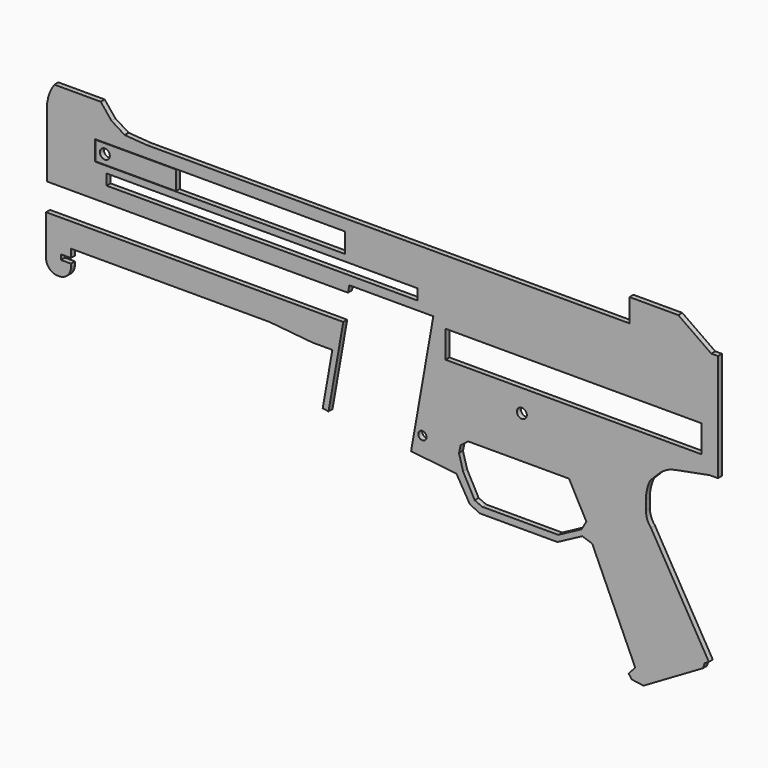
from build123d import *

# Parameters (mm, degrees)
F0_R     = 2.5
F0_W     = 187.8374901577
F0_H     = 6.5
F0_W_2   = 151
F0_H_2   = 12
F0_R_2   = 3
F0_W_3   = 154.6288044202
F0_H_3   = 16.5
F1_DEPTH = 3
F0_W_4   = 48.75
F0_H_4   = 11.5


with BuildPart() as f1:
    # F0 (on Front) → F1 (new body)
    with BuildSketch(Plane.XZ):
        with BuildLine():
            Line((48.5, -65), (53.5, -65))
            Line((53.5, -65), (53.5, 0))
            Line((53.5, 0), (49.5, 0))
            Line((49.5, 0), (29.55, 14))
            Line((29.55, 14), (0, 14))
            Line((0, 14), (0, 0))
            Line((0, 0), (-291.5, 0))
            Line((-291.5, 0), (-305, 1))
            Line((-305, 1), (-313, 6))
            Line((-313, 6), (-319.5, 14))
            Line((-319.5, 14), (-347.5, 14))
            ThreePointArc((-347.5, 14), (-350.8473529309, 7.3527205849), (-352, 0))
            Line((-352, 0), (-352, -39))
            Line((-352, -39), (-170.0255081496, -39))
            Line((-170.0255081496, -39), (-169.2796367248, -34.7699529486))
            Line((-169.2796367248, -34.7699529486), (-118.5083061305, -34.7699529486))
            Line((-118.5083061305, -34.7699529486), (-119.2130711177, -38.7668738074))
            Line((-119.2130711177, -38.7668738074), (-122.163572737, -55.5))
            Line((-122.163572737, -55.5), (-131.940312204, -110.9466447942))
            Line((-131.940312204, -110.9466447942), (-104.5, -114))
            Line((-104.5, -114), (-96.5, -127.5))
            Line((-96.5, -127.5), (-90.5, -130.5))
            Line((-90.5, -130.5), (-43.5, -130.5))
            Line((-43.5, -130.5), (-28.5, -122.5))
            Line((-28.5, -122.5), (-22.5, -124.5))
            Line((-22.5, -124.5), (3.5, -182))
            Line((3.5, -182), (-0.5, -186.5))
            Line((-0.5, -186.5), (1.5, -189))
            Line((1.5, -189), (8.5, -190))
            Line((8.5, -190), (44.5, -169))
            Line((44.5, -169), (45.5, -166))
            Line((45.5, -166), (48, -164.5))
            Line((48, -164.5), (13, -104.5))
            ThreePointArc((13, -104.5), (10.7746616729, -100.7720018727), (10, -96.5))
            Line((10, -96.5), (10, -90.5))
            ThreePointArc((10, -90.5), (10.6328688201, -84.8597429137), (12.5, -79.5))
            Line((12.5, -79.5), (18.5, -73.5))
            ThreePointArc((18.5, -73.5), (22.688171875, -70.6263437501), (27.5, -69))
            Line((27.5, -69), (48.5, -65))
        make_face()
        with Locations((-125.101, -100.41)):
            Circle(F0_R, mode=Mode.SUBTRACT)
        Polygon((-36.5, -94.5), (-26, -114), (-29, -119), (-43, -126.5), (-89, -126.5), (-93.5, -124.5), (-100.5, -111.5), (-103, -102.5), (-102, -98), (-97.5, -94.5), align=None, mode=Mode.SUBTRACT)
        with Locations((-222.0812549212, -26.25)):
            Rectangle(F0_W, F0_H, mode=Mode.SUBTRACT)
        with Locations((-247.5, -13)):
            Rectangle(F0_W_2, F0_H_2, mode=Mode.SUBTRACT)
        with Locations((-65, -69)):
            Circle(F0_R_2, mode=Mode.SUBTRACT)
        with Locations((-33.8144022101, -47.25)):
            Rectangle(F0_W_3, F0_H_3, mode=Mode.SUBTRACT)
    extrude(amount=F1_DEPTH)


with BuildPart() as f1b:
    # F0 (on Front) → F1, piece 2 (new body)
    with BuildSketch(Plane.XZ):
        with BuildLine():
            ThreePointArc((-352.5206254937, -80), (-350.470372962, -84.9497474683), (-345.5206254937, -87))
            Line((-345.5206254937, -87), (-344.5206254937, -87))
            ThreePointArc((-344.5206254937, -87), (-339.5708780254, -84.9497474683), (-337.5206254937, -80))
            Line((-337.5206254937, -80), (-337.5206254937, -78))
            Line((-337.5206254937, -78), (-343.5206254937, -78))
            Line((-343.5206254937, -78), (-343.5206254937, -75))
            Line((-343.5206254937, -75), (-337.5206254937, -75))
            Line((-337.5206254937, -75), (-337.5206254937, -70))
            Line((-337.5206254937, -70), (-217.5206254937, -70))
            Line((-217.5206254937, -70), (-191.5206254937, -72.5))
            Line((-191.5206254937, -72.5), (-179.5206254937, -72.5))
            Line((-179.5206254937, -72.5), (-185.3394158571, -105.5))
            Line((-185.3394158571, -105.5), (-181.8394158571, -106))
            Line((-181.8394158571, -106), (-172.9349033313, -55.5))
            Line((-172.9349033313, -55.5), (-352.5206254937, -55.5))
            Line((-352.5206254937, -55.5), (-352.5206254937, -80))
        make_face()
    extrude(amount=F1_DEPTH)


with BuildPart() as f1c:
    # F0 (on Front) → F1, piece 3 (new body)
    with BuildSketch(Plane.XZ):
        with Locations((-298.375, -13)):
            Rectangle(F0_W_4, F0_H_4)
        with Locations((-317, -13)):
            Circle(F0_R_2, mode=Mode.SUBTRACT)
    extrude(amount=F1_DEPTH)


solid = Compound([f1.part, f1b.part, f1c.part])
